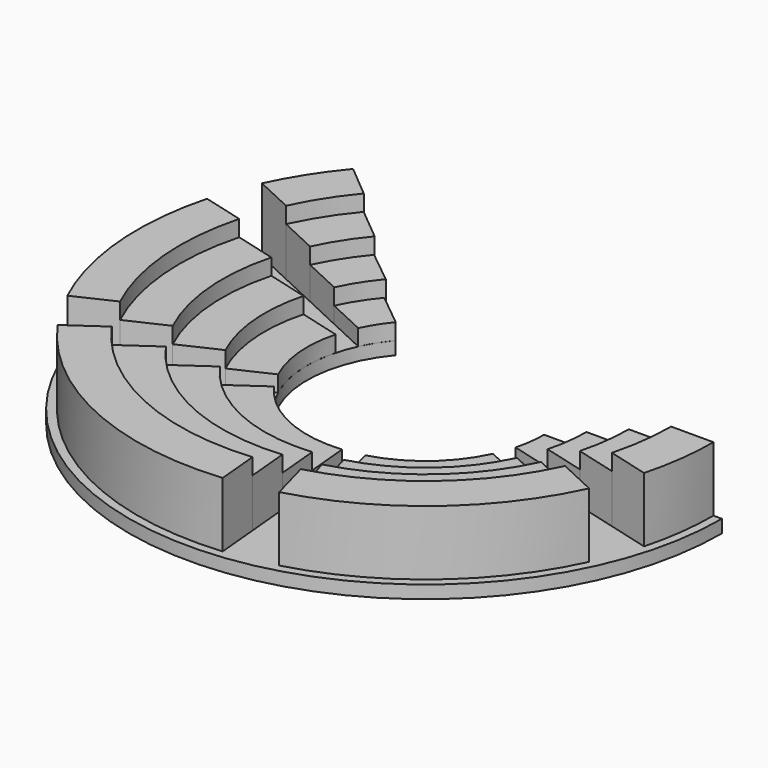
from build123d import *

# Parameters (mm, degrees)
F0_W      = 91.66666
F0_H      = 4
F1_ANGLE  = 220
F2_R      = 36.666665
F3_DEPTH  = 12.5
F5_DEPTH  = 5
F7_DEPTH  = 10
F9_DEPTH  = 15
F11_DEPTH = 20
F13_DEPTH = 29
F15_DEPTH = 25


with BuildPart() as f1:
    # F0 (on Front) → F1 (revolve)
    with BuildSketch(Plane.XZ):
        with Locations((45.83333, -2)):
            Rectangle(F0_W, F0_H)
    revolve(axis=Axis((0, 0, -2), (0, 0, -1)), revolution_arc=F1_ANGLE)

    # F2 (on Top) → F3 (cut, symmetric)
    with BuildSketch(Plane.XY):
        Circle(F2_R)
    extrude(amount=F3_DEPTH, both=True, mode=Mode.SUBTRACT)


with BuildPart() as f5:
    # F4 (on Top) → F5 (new body)
    with BuildSketch(Plane.XY):
        with BuildLine():
            ThreePointArc((36.6666665, 0), (-12.540655641, -34.4554261085), (-28.0884095207, 23.5687437684))
            Line((-28.0884095207, 23.5687437684), (-38.2522682412, 31.827203092))
            ThreePointArc((-38.2522682412, 31.827203092), (-16.9221251054, -46.7958178064), (49.7615, 0))
            Line((49.7615, 0), (36.6666665, 0))
        make_face()
    extrude(amount=F5_DEPTH)


with BuildPart() as f7:
    # F6 (on Top) → F7 (new body)
    with BuildSketch(Plane.XY):
        with BuildLine():
            ThreePointArc((49.7615, 0), (-17.1048840177, -46.7293251074), (-38.0023264518, 32.1252247696))
            Line((-38.0023264518, 32.1252247696), (-48.2022163099, 40.3431239363))
            ThreePointArc((-48.2022163099, 40.3431239363), (-21.4612134466, -59.0799257237), (62.85715, 0))
            Line((62.85715, 0), (49.7615, 0))
        make_face()
    extrude(amount=F7_DEPTH)


with BuildPart() as f9:
    # F8 (on Top) → F9 (new body)
    with BuildSketch(Plane.XY):
        with BuildLine():
            Line((-48.1102146254, 40.452778615), (-58.190830552, 48.8118254671))
            ThreePointArc((-58.190830552, 48.8118254671), (-25.9714634488, -71.3740159448), (75.9524, 0))
            Line((75.9524, 0), (62.85714, 0))
            ThreePointArc((62.85714, 0), (-21.5284643303, -59.0554423619), (-48.1102146254, 40.452778615))
        make_face()
    extrude(amount=F9_DEPTH)


with BuildPart() as f11:
    # F10 (on Top) → F11 (new body)
    with BuildSketch(Plane.XY):
        with BuildLine():
            ThreePointArc((75.95235, 0), (-25.9780129339, -71.3715791792), (-58.1818094968, 48.8225000814))
            Line((-58.1818094968, 48.8225000814), (-68.2119472637, 57.2416397061))
            ThreePointArc((-68.2119472637, 57.2416397061), (-30.4578796914, -83.6767149837), (89.0476, 0))
            Line((89.0476, 0), (75.95235, 0))
        make_face()
    extrude(amount=F11_DEPTH)


with BuildPart() as f13_tool:
    # F12 (on Top) → F13 (new body)
    with BuildSketch(Plane.XY):
        Polygon((94.6472080148, -25.3606429534), (0, 0), (88.5066497486, -41.2713285754), align=None)
        Polygon((-94.3287258626, 25.2753059179), (0, 0), (-88.8055123304, 41.4106904861), align=None)
    extrude(amount=F13_DEPTH)


with BuildPart() as f5_1:
    add(f5.part)

    # F13: cut by f13_tool
    add(f13_tool.part, mode=Mode.SUBTRACT)


with BuildPart() as f7_1:
    add(f7.part)

    # F13: cut by f13_tool
    add(f13_tool.part, mode=Mode.SUBTRACT)


with BuildPart() as f9_1:
    add(f9.part)

    # F13: cut by f13_tool
    add(f13_tool.part, mode=Mode.SUBTRACT)


with BuildPart() as f11_1:
    add(f11.part)

    # F13: cut by f13_tool
    add(f13_tool.part, mode=Mode.SUBTRACT)


with BuildPart() as f15_tool:
    # F14 (on Top) → F15 (new body)
    with BuildSketch(Plane.XY):
        Polygon((-80.2769003403, -56.2104907624), (0, 0), (-88.8181631296, -41.4165896506), align=None)
        Polygon((25.0542324687, -91.7911742938), (0, 0), (8.8207321241, -95.6856161356), align=None)
    extrude(amount=F15_DEPTH)


with BuildPart() as f5_2:
    add(f5_1.part)

    # F15: cut by f15_tool
    add(f15_tool.part, mode=Mode.SUBTRACT)


with BuildPart() as f7_2:
    add(f7_1.part)

    # F15: cut by f15_tool
    add(f15_tool.part, mode=Mode.SUBTRACT)


with BuildPart() as f9_2:
    add(f9_1.part)

    # F15: cut by f15_tool
    add(f15_tool.part, mode=Mode.SUBTRACT)


with BuildPart() as f11_2:
    add(f11_1.part)

    # F15: cut by f15_tool
    add(f15_tool.part, mode=Mode.SUBTRACT)


solid = Compound([f1.part, f5_2.part, f7_2.part, f9_2.part, f11_2.part])
